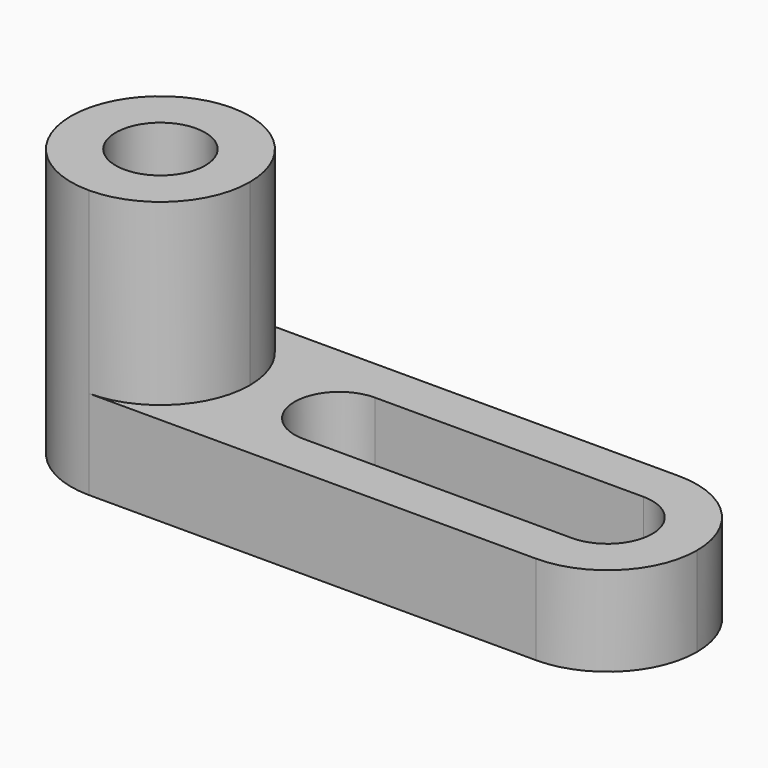
from build123d import *

# Parameters (mm, degrees)
F0_W     = 88.9
F0_H     = 12.7
F1_DEPTH = 25.4
F2_R     = 6.35
F3_DEPTH = 25.4
F4_DEPTH = 62.23
F6_DEPTH = 25.4
F8_DEPTH = 25.4
F9_DEPTH = 25.4


with BuildPart() as f1:
    # F0 (on Front) → F1 (new body)
    with BuildSketch(Plane.XZ):
        with Locations((44.45, 6.35)):
            Rectangle(F0_W, F0_H)
    extrude(amount=-F1_DEPTH)

    # F2 (on face) → F3 (join)
    with BuildSketch(Plane.XY.offset(12.7)):
        with BuildLine():
            ThreePointArc((12.7, 0), (21.680256, 3.719744), (25.4, 12.7))
            ThreePointArc((25.4, 12.7), (21.680256, 21.680256), (12.7, 25.4))
            ThreePointArc((12.7, 25.4), (3.719744, 21.680256), (0, 12.7))
            ThreePointArc((0, 12.7), (3.719744, 3.719744), (12.7, 0))
        make_face()
        with Locations((12.7, 12.7)):
            Circle(F2_R, mode=Mode.SUBTRACT)
    extrude(amount=F3_DEPTH)

    # F4 (cut): faces of the model
    f4_faces = [f1.faces().sort_by_distance(p)[0] for p in [
        (2.836773, 22.563227, 12.7),
        (2.836773, 2.836773, 12.7),
    ]]
    extrude(f4_faces, amount=-F4_DEPTH, mode=Mode.SUBTRACT)

    # F5 (on face) → F6 (cut)
    with BuildSketch(Plane.XY.offset(12.7)):
        with BuildLine():
            Line((76.2, 19.05), (38.1, 19.05))
            ThreePointArc((38.1, 19.05), (31.75, 12.7), (38.1, 6.35))
            Line((38.1, 6.35), (76.2, 6.35))
            ThreePointArc((76.2, 6.35), (82.55, 12.7), (76.2, 19.05))
        make_face()
    extrude(amount=-F6_DEPTH, mode=Mode.SUBTRACT)

    # F7 (on face) → F8 (cut)
    with BuildSketch(Plane.XY.offset(12.7)):
        with BuildLine():
            ThreePointArc((76.2, 25.4), (85.180256, 21.680256), (88.9, 12.7))
            Line((88.9, 12.7), (88.9, 25.4))
            Line((88.9, 25.4), (76.2, 25.4))
        make_face()
        with BuildLine():
            ThreePointArc((88.9, 12.7), (85.180256, 3.719744), (76.2, 0))
            Line((76.2, 0), (88.9, 0))
            Line((88.9, 0), (88.9, 12.7))
        make_face()
    extrude(amount=-F8_DEPTH, mode=Mode.SUBTRACT)

    # F9 (cut): a face of the model
    f9_faces = [f1.faces().sort_by_distance(p)[0] for p in [
        (12.7, 12.7, 12.7),
    ]]
    extrude(f9_faces, amount=-F9_DEPTH, mode=Mode.SUBTRACT)


solid = f1.part
